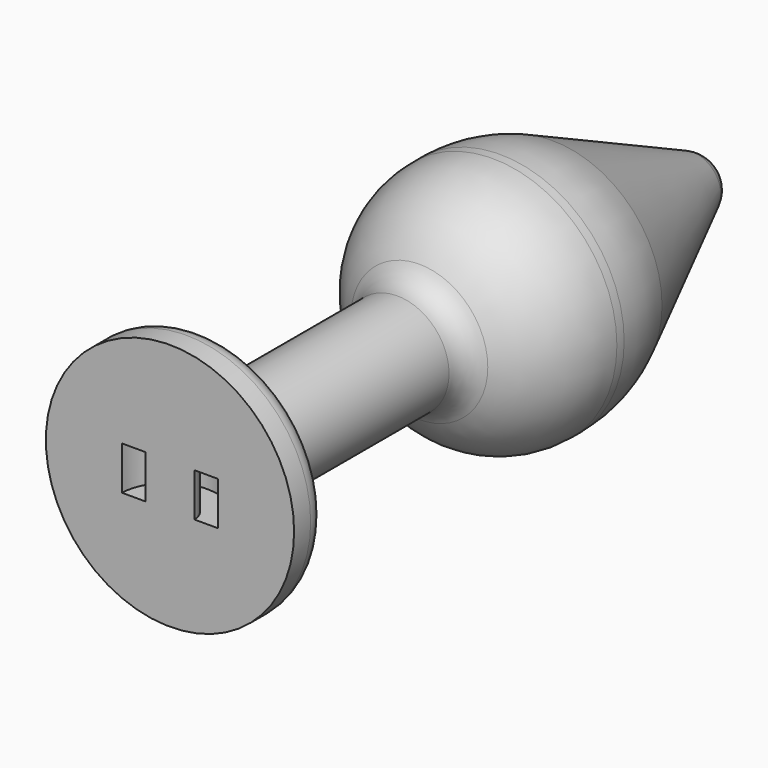
from build123d import *

# Parameters (mm, degrees)
F2_R     = 2
F3_R     = 2
F4_R     = 4.6529317806
F4_R_2   = 2.3810630886
F5_DEPTH = 2.1


# Not quite as in the source:
# - a feature names something its author has since deleted; it is built from what else it names


with BuildPart() as f1:
    # F0 (on Top) → F1 (revolve)
    with BuildSketch(Plane.XY):
        with BuildLine():
            Line((12, 0), (5, 0))
            Line((5, 0), (5, 23.4674374053))
            ThreePointArc((5, 23.4674374053), (5.4354487572, 25.0240609703), (6.6153846154, 26.1287980041))
            ThreePointArc((6.6153846154, 26.1287980041), (10.5485041427, 29.8112547834), (12, 35))
            Line((12, 35), (12, 35.8777977526))
            ThreePointArc((12, 35.8777977526), (11.6461494723, 39.1166718836), (10.6012925819, 42.2027357051))
            Line((10.6012925819, 42.2027357051), (2.7202585164, 59.1502932902))
            ThreePointArc((2.7202585164, 59.1502932902), (1.6132323497, 60.414629994), (0, 60.8853056997))
            Line((0, 60.8853056997), (0, 25))
            Line((0, 25), (0, 17.2050446272))
            Line((0, 17.2050446272), (0, -4))
            Line((0, -4), (9, -4))
            Line((9, -4), (12, -4))
            Line((12, -4), (12, 0))
        make_face()
    revolve(axis=Axis((0, 21.1025223136, 0), (0, -1, 0)))

    # F2
    f2_edges = [f1.edges().sort_by_distance(p)[0] for p in [
        (-12, 0, 0),
    ]]
    fillet(f2_edges, radius=F2_R)

    # F3
    f3_edges = [f1.edges().sort_by_distance(p)[0] for p in [
        (-5, 0, 0),
    ]]
    fillet(f3_edges, radius=F3_R)

    # F4 (on Top) → F5 (cut, symmetric)
    with BuildSketch(Plane.XY):
        with Locations((0, -4.1621848941)):
            Circle(F4_R)
        with Locations((0, -4.1621848941)):
            Circle(F4_R_2, mode=Mode.SUBTRACT)
    extrude(amount=F5_DEPTH, both=True, mode=Mode.SUBTRACT)


solid = f1.part
